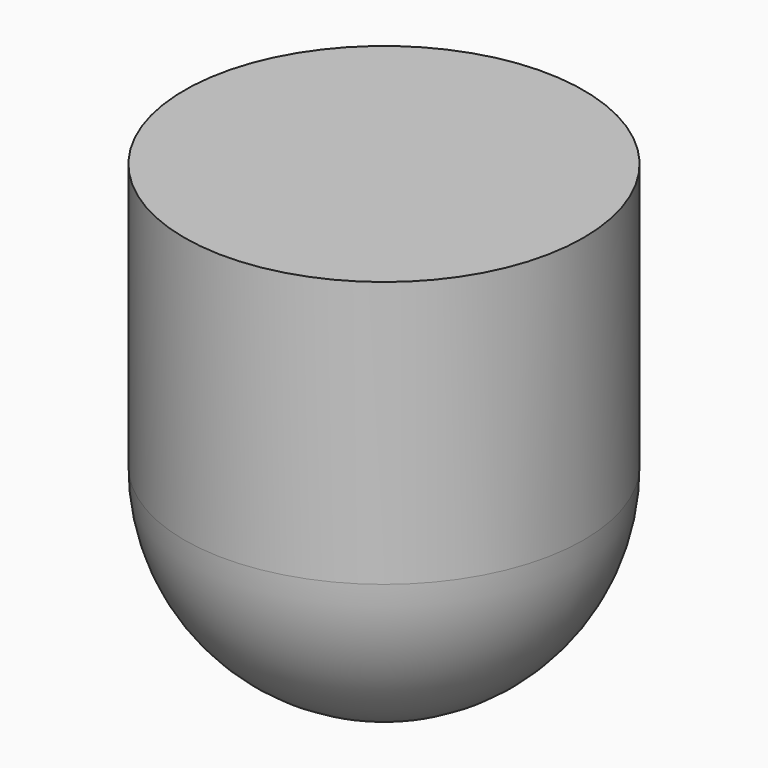
from build123d import *

# Parameters (mm, degrees)
F0_W = 30
F0_H = 40


# Not quite as in the source:
# - a feature names something its author has since deleted; it is built from what else it names


with BuildPart() as f1:
    # F0 (on Front) → F1 (revolve)
    with BuildSketch(Plane.XZ):
        with Locations((15, 50)):
            Rectangle(F0_W, F0_H)
        with BuildLine():
            Line((30, 30), (0, 30))
            Line((0, 30), (0, 0))
            ThreePointArc((0, 0), (21.2132034356, 8.7867965644), (30, 30))
        make_face()
    revolve(axis=Axis((0, 0, 50), (0, 0, -1)))


solid = f1.part
